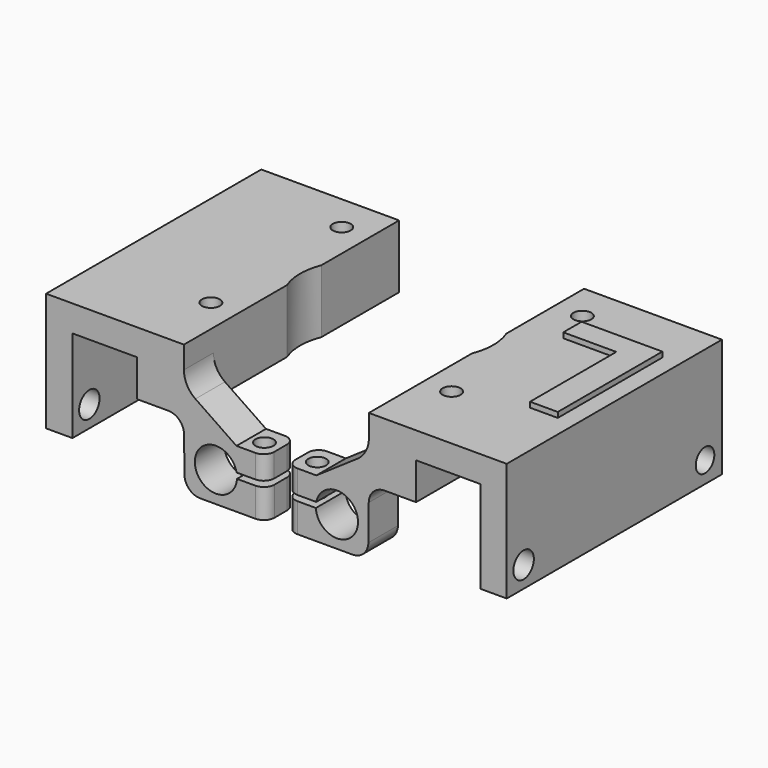
from build123d import *

# Parameters (mm, degrees)
F1_DEPTH      = 7
F2_DEPTH      = 44
F3_R          = 1.7
F3_R_2        = 11
F4_DEPTH      = 12.001
F5_R          = 4
F6_DEPTH      = 10
F7_DEPTH      = 12.001
F8_R          = 1.4
F9_DEPTH      = 10.9920075553
F8_R_2        = 1.7
F10_DEPTH     = 4.4348209087
F11_R         = 5
F12_R         = 3
F13_R         = 3
F14_R         = 2
F15_R         = 2.2
F15_R_2       = 2.4255023423
F16_DEPTH     = 6
F19_TEXT_SIZE = 34.7222222222
F20_DEPTH     = 1


# Not quite as in the source:
# - a feature names something its author has since deleted; it is built from what else it names
# - Text() gives the source's letters only with a copy of the font that has no kerning and outlines rounded to 1/6400 em; it was checked with that copy


with BuildPart() as f1:
    # F0 (on Front) → F1 (new body)
    with BuildSketch(Plane.XZ):
        Polygon((-18.6721007523, 29.8099789735), (-18.6721007523, 7.3259699669), (-13.6721007523, 7.3259699669), (-13.6721007523, 24.8099789735), (-1.4721007523, 24.8099789735), (-1.4721007523, 17.8099789735), (7.4637966118, 17.8099789735), (7.4637966118, 22.9406704692), (7.4637966118, 29.8099789735), align=None)
        Polygon((17.4301751077, 16.1394868046), (7.4637966118, 22.9406704692), (7.4637966118, 17.8099789735), (7.5940201178, 5.1484792493), (23.0186601057, 5.1484792493), (23.0186601057, 10.6682249423), (15.6860510706, 10.6682249423), (15.6860510706, 11.7046658959), (22.9896428882, 11.7046658959), (22.9896428882, 16.1394868046), align=None)
    extrude(amount=F1_DEPTH)

    # F0 (on Front) → F2 (join)
    with BuildSketch(Plane.XZ):
        Polygon((-18.6721007523, 29.8099789735), (-18.6721007523, 7.3259699669), (-13.6721007523, 7.3259699669), (-13.6721007523, 24.8099789735), (-1.4721007523, 24.8099789735), (-1.4721007523, 17.8099789735), (7.4637966118, 17.8099789735), (7.4637966118, 22.9406704692), (7.4637966118, 29.8099789735), align=None)
    extrude(amount=-F2_DEPTH)

    # F3 (on face) → F4 (cut, through all)
    with BuildSketch(Plane(origin=(0, 0, 17.8099789735), x_dir=(1, 0, 0), z_dir=(0, 0, -1))):
        with Locations((2.1850741468, -6)):
            Circle(F3_R)
        with Locations((2.1850741468, -37)):
            Circle(F3_R)
        with Locations((17.6850741468, -21.5)):
            Circle(F3_R_2)
    extrude(amount=-F4_DEPTH, mode=Mode.SUBTRACT)

    # F5 (on face) → F6 (cut)
    with BuildSketch(Plane.XZ.offset(7)):
        with Locations((13.5278992477, 10.8989789735)):
            Circle(F5_R)
    extrude(amount=-F6_DEPTH, mode=Mode.SUBTRACT)

    # F3 (on face) → F7 (cut, through all)
    with BuildSketch(Plane(origin=(0, 0, 17.8099789735), x_dir=(1, 0, 0), z_dir=(0, 0, -1))):
        with Locations((2.1850741468, -6)):
            Circle(F3_R)
        with Locations((2.1850741468, -37)):
            Circle(F3_R)
        with Locations((17.6850741468, -21.5)):
            Circle(F3_R_2)
    extrude(amount=-F7_DEPTH, mode=Mode.SUBTRACT)

    # F8 (on face) → F9 (cut, through all)
    with BuildSketch(Plane.XY.offset(16.1394868046)):
        with Locations((19.9896428882, -3.5767070949)):
            Circle(F8_R)
    extrude(amount=-F9_DEPTH, mode=Mode.SUBTRACT)

    # F8 (on face) → F10 (cut, through all)
    with BuildSketch(Plane.XY.offset(16.1394868046)):
        with Locations((19.9896428882, -3.5767070949)):
            Circle(F8_R_2)
        with Locations((19.9896428882, -3.5767070949)):
            Circle(F8_R, mode=Mode.SUBTRACT)
    extrude(amount=-F10_DEPTH, mode=Mode.SUBTRACT)

    # F11
    f11_edges = [f1.edges().sort_by_distance(p)[0] for p in [
        (7.463797, -3.5, 22.94067),
    ]]
    fillet(f11_edges, radius=F11_R)

    # F12
    f12_edges = [f1.edges().sort_by_distance(p)[0] for p in [
        (7.463797, -3.5, 17.809979),
    ]]
    fillet(f12_edges, radius=F12_R)

    # F13
    f13_edges = [f1.edges().sort_by_distance(p)[0] for p in [
        (7.59402, -3.5, 5.148479),
    ]]
    fillet(f13_edges, radius=F13_R)

    # F14
    f14_edges = [f1.edges().sort_by_distance(p)[0] for p in [
        (22.989643, -7, 13.922076),
        (23.01866, -7, 7.908352),
        (22.989643, 0, 13.922076),
        (23.01866, 0, 7.908352),
    ]]
    fillet(f14_edges, radius=F14_R)

    # F15 (on face) → F16 (cut)
    with BuildSketch(Plane(origin=(-18.6721007523, 0, 0), x_dir=(0, -1, 0), z_dir=(-1, 0, 0))):
        with Locations((-40, 11.3259699669)):
            Circle(F15_R)
        with Locations((3, 11.3259699669)):
            Circle(F15_R_2)
    extrude(amount=-F16_DEPTH, mode=Mode.SUBTRACT)


with BuildPart() as f17_1:
    # F17: instance of F1
    add(f1.part.mirror(Plane.YZ))


with BuildPart() as f17_1_1:
    # F18: moved
    add(f17_1.part.moved(Location((50, 0, 0))))

    # F19 (on face) → F20 (join)
    with BuildSketch(Plane.XY.offset(29.8099789735)):
        with Locations(Location((68.4963494643, 34), (0, 0, 180))):
            Text('L', F19_TEXT_SIZE, font='Open Sans', font_style=FontStyle.BOLD, text_align=(TextAlign.LEFT, TextAlign.BOTTOM))
    extrude(amount=F20_DEPTH)


solid = Compound([f1.part, f17_1_1.part])
